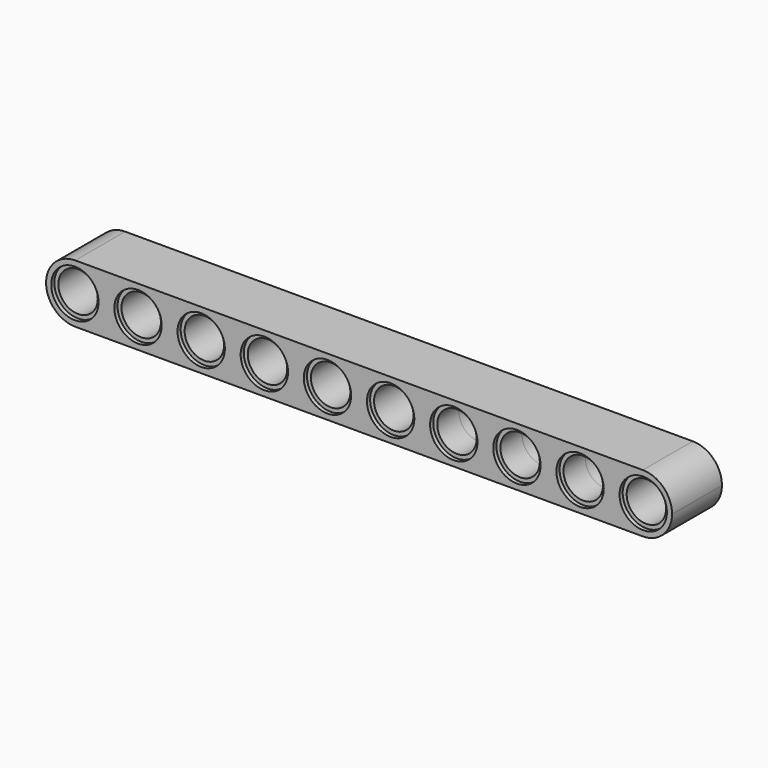
from build123d import *

# Parameters (mm, degrees)
F0_R     = 3
F1_DEPTH = 3.95
F0_R_2   = 2.499
F0_R_3   = 2.495
F2_DEPTH = 3.45
F3_R     = 3.69999
F4_R     = 3.69999


# Not quite as in the source:
# - a fillet or chamfer is up to 0.001 mm smaller than in the source, because OpenCascade refuses the exact size


with BuildPart() as f1:
    # F0 (on Front) → F1 (new body, symmetric)
    with BuildSketch(Plane.XZ):
        Polygon((-39.65, 3.7), (-39.65, -3.7), (39.65, -3.7), (39.65, 3.7), (0, 3.7), align=None)
        with Locations((-36, 0)):
            Circle(F0_R, mode=Mode.SUBTRACT)
        with Locations((-28, 0)):
            Circle(F0_R, mode=Mode.SUBTRACT)
        with Locations((-20, 0)):
            Circle(F0_R, mode=Mode.SUBTRACT)
        with Locations((-12, 0)):
            Circle(F0_R, mode=Mode.SUBTRACT)
        with Locations((-4, 0)):
            Circle(F0_R, mode=Mode.SUBTRACT)
        with BuildLine():
            ThreePointArc((7, 0), (4, -3), (1, 0))
            ThreePointArc((1, 0), (4, 3), (7, 0))
        make_face(mode=Mode.SUBTRACT)
        with Locations((12, 0)):
            Circle(F0_R, mode=Mode.SUBTRACT)
        with Locations((20, 0)):
            Circle(F0_R, mode=Mode.SUBTRACT)
        with Locations((28, 0)):
            Circle(F0_R, mode=Mode.SUBTRACT)
        with Locations((36, 0)):
            Circle(F0_R, mode=Mode.SUBTRACT)
    extrude(amount=F1_DEPTH, both=True)

    # F0 (on Front) → F2 (join, symmetric)
    with BuildSketch(Plane.XZ):
        with Locations((-36, 0)):
            Circle(F0_R)
        with Locations((-36, 0)):
            Circle(F0_R_2, mode=Mode.SUBTRACT)
        with Locations((-28, 0)):
            Circle(F0_R)
        with Locations((-28, 0)):
            Circle(F0_R_2, mode=Mode.SUBTRACT)
        with Locations((-20, 0)):
            Circle(F0_R)
        with Locations((-20, 0)):
            Circle(F0_R_2, mode=Mode.SUBTRACT)
        with Locations((-12, 0)):
            Circle(F0_R)
        with Locations((-12, 0)):
            Circle(F0_R_2, mode=Mode.SUBTRACT)
        with Locations((-4, 0)):
            Circle(F0_R)
        with Locations((-4, 0)):
            Circle(F0_R_2, mode=Mode.SUBTRACT)
        with BuildLine():
            ThreePointArc((7, 0), (4, 3), (1, 0))
            ThreePointArc((1, 0), (4, -3), (7, 0))
        make_face()
        with BuildLine():
            ThreePointArc((6.499, 0), (4, -2.499), (1.501, 0))
            ThreePointArc((1.501, 0), (4, 2.499), (6.499, 0))
        make_face(mode=Mode.SUBTRACT)
        with Locations((12, 0)):
            Circle(F0_R)
        with Locations((12, 0)):
            Circle(F0_R_3, mode=Mode.SUBTRACT)
        with Locations((20, 0)):
            Circle(F0_R)
        with Locations((20, 0)):
            Circle(F0_R_2, mode=Mode.SUBTRACT)
        with Locations((28, 0)):
            Circle(F0_R)
        with Locations((28, 0)):
            Circle(F0_R_2, mode=Mode.SUBTRACT)
        with Locations((36, 0)):
            Circle(F0_R)
        with Locations((36, 0)):
            Circle(F0_R_2, mode=Mode.SUBTRACT)
    extrude(amount=F2_DEPTH, both=True)

    # F3 (radius 3.7 in the source; OpenCascade refuses exactly that, so slightly less here)
    f3_edges = [f1.edges().sort_by_distance(p)[0] for p in [
        (39.65, 0, 3.7),
        (39.65, 0, -3.7),
    ]]
    fillet(f3_edges, radius=F3_R)

    # F4 (radius 3.7 in the source; OpenCascade refuses exactly that, so slightly less here)
    f4_edges = [f1.edges().sort_by_distance(p)[0] for p in [
        (-39.65, 0, 3.7),
        (-39.65, 0, -3.7),
    ]]
    fillet(f4_edges, radius=F4_R)


solid = f1.part
